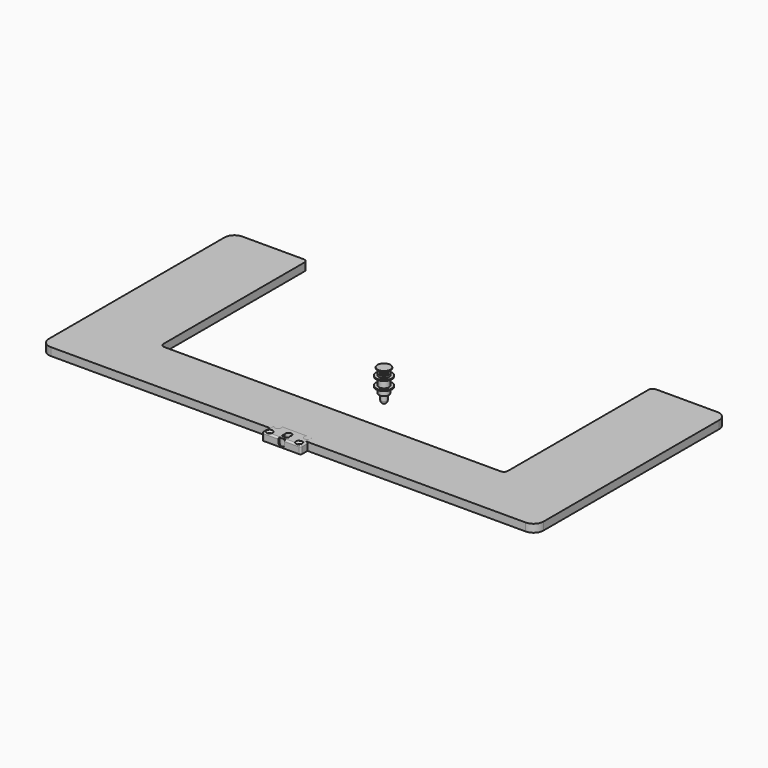
from build123d import *

# Parameters (mm, degrees)
F0_R           = 8.0391
F1_DEPTH       = 12.7
F2_W           = 62.0164461434
F2_H           = 28.0967354774
F2_R           = 4.8895
F3_DEPTH       = 12.7
F7_R           = 2.54
F9_D           = 4.7498
F9_CSINK_D     = 10.16
F9_CSINK_ANGLE = 82
F10_W          = 4.7498
F10_H          = 1.6002


with BuildPart() as f1:
    # F0 (on Top) → F1 (new body)
    with BuildSketch(Plane.XY):
        with BuildLine():
            ThreePointArc((-396.8930379433, -176.0628120543), (-392.25524501, -187.3556160105), (-381.0191923747, -192.1292588187))
            Line((-381.0191923747, -192.1292588187), (-29.9185505861, -192.1292588187))
            ThreePointArc((-29.9185505861, -192.1292588187), (-28.4575333665, -192.2996205863), (-27.0749103125, -192.801564745))
            Line((-27.0749103125, -192.801564745), (-5.7064793941, -203.503819913))
            ThreePointArc((-5.7064793941, -203.503819913), (-0.0095961873, -204.8507020685), (5.6872870194, -203.503819913))
            Line((5.6872870194, -203.503819913), (27.0557179378, -192.801564745))
            ThreePointArc((27.0557179378, -192.801564745), (28.4383409918, -192.2996205863), (29.8993582114, -192.1292588187))
            Line((29.8993582114, -192.1292588187), (381, -192.1292588187))
            ThreePointArc((381, -192.1292588187), (392.2253201513, -187.4795789701), (396.875, -176.2542588187))
            Line((396.875, -176.2542588187), (396.875, 176.1707411813))
            ThreePointArc((396.875, 176.1707411813), (392.2253201513, 187.3960613326), (381, 192.0457411813))
            Line((381, 192.0457411813), (282.575, 192.0457411813))
            ThreePointArc((282.575, 192.0457411813), (278.0848719395, 190.1858692418), (276.225, 185.6957411813))
            Line((276.225, 185.6957411813), (276.225, -96.8792588187))
            ThreePointArc((276.225, -96.8792588187), (274.3651280605, -101.3693868793), (269.875, -103.2292588187))
            Line((269.875, -103.2292588187), (-269.8930379433, -103.2292588187))
            ThreePointArc((-269.8930379433, -103.2292588187), (-274.3831660038, -101.3693868793), (-276.2430379433, -96.8792588187))
            Line((-276.2430379433, -96.8792588187), (-276.2430379433, 185.6957411813))
            ThreePointArc((-276.2430379433, 185.6957411813), (-278.1029098828, 190.1858692418), (-282.5930379433, 192.0457411813))
            Line((-282.5930379433, 192.0457411813), (-381.0180379433, 192.0457411813))
            ThreePointArc((-381.0180379433, 192.0457411813), (-392.2433580946, 187.3960613326), (-396.8930379433, 176.1707411813))
            Line((-396.8930379433, 176.1707411813), (-396.8930379433, -176.0628120543))
        make_face()
        with Locations((-0.0095961873, -192.1292588187)):
            Circle(F0_R, mode=Mode.SUBTRACT)
    extrude(amount=F1_DEPTH)


with BuildPart() as f3:
    # F2 (on Top) → F3 (new body)
    with BuildSketch(Plane.XY):
        with Locations((0, -191.5318369865)):
            Rectangle(F2_W, F2_H)
        with Locations((0, -191.5318369865)):
            Circle(F2_R, mode=Mode.SUBTRACT)
    extrude(amount=F3_DEPTH)

    # F6: sweep along a path in F4
    with BuildLine(Plane.YZ) as f6_path:
        Line((-205.5802047253, 2.0510469544), (-192.8892766759, 12.7))
    # F5 (on face) → F6 (sweep, cut)
    with BuildSketch(Plane.XZ.offset(205.5802047253)):
        with BuildLine():
            Line((-4.7625, 12.7), (-4.7625, 5.3647807799))
            ThreePointArc((-4.7625, 5.3647807799), (0, 0.6022807799), (4.7625, 5.3647807799))
            Line((4.7625, 5.3647807799), (4.7625, 12.7))
            Line((4.7625, 12.7), (-4.7625, 12.7))
        make_face()
    sweep(path=f6_path.line, mode=Mode.SUBTRACT)

    # F7
    f7_edges = [f3.edges().sort_by_distance(p)[0] for p in [
        (-31.008223, -191.531837, 12.7),
        (-17.885362, -205.580205, 12.7),
        (17.885362, -205.580205, 12.7),
        (31.008223, -191.531837, 12.7),
        (0, -177.483469, 12.7),
        (31.008223, -205.580205, 6.35),
        (31.008223, -177.483469, 6.35),
        (-31.008223, -205.580205, 6.35),
        (-31.008223, -177.483469, 6.35),
    ]]
    fillet(f7_edges, radius=F7_R)

    # F9 (through all)
    with Locations(Plane.XY.offset(12.7)):
        with Locations((-23.5967673361, -183.2025200129), (23.5967673361, -183.2025200129), (23.5967673361, -199.8611539602), (-23.5967673361, -199.8611539602)):
            CounterSinkHole(F9_D / 2, F9_CSINK_D / 2, counter_sink_angle=F9_CSINK_ANGLE)


with BuildPart() as f11:
    # F10 (on Front) → F11 (revolve)
    with BuildSketch(Plane.XZ):
        with BuildLine():
            ThreePointArc((0, -21.0152691894), (3.3675960454, -19.6203652348), (4.7625, -16.2527691894))
            Line((4.7625, -16.2527691894), (4.7625, -6.796184157))
            Line((4.7625, -6.796184157), (7.9375, -6.796184157))
            Line((7.9375, -6.796184157), (7.9375, 2.7130942824))
            Line((7.9375, 2.7130942824), (7.9375, 4.3132942824))
            Line((7.9375, 4.3132942824), (7.9375, 17.0132942824))
            Line((7.9375, 17.0132942824), (7.9375, 18.6134942824))
            Line((7.9375, 18.6134942824), (7.9375, 21.7884942824))
            Line((7.9375, 21.7884942824), (5.08, 21.7884942824))
            Line((5.08, 21.7884942824), (5.08, 23.7518632694))
            Line((5.08, 23.7518632694), (10.414, 28.596999448))
            Line((10.414, 28.596999448), (10.414, 30.1022308106))
            Line((10.414, 30.1022308106), (0, 30.1022308106))
            Line((0, 30.1022308106), (0, -21.0152691894))
        make_face()
    revolve(axis=Axis((0, 0, 4.5434808106), (0, 0, -1)))


with BuildPart() as f12:
    # F10 (on Front) → F12 (revolve)
    with BuildSketch(Plane.XZ):
        with Locations((10.3124, 17.8133942824)):
            Rectangle(F10_W, F10_H)
    revolve(axis=Axis((0, 0, 4.5434808106), (0, 0, -1)))


with BuildPart() as f12b:
    # F10 (on Front) → F12, piece 2 (revolve)
    with BuildSketch(Plane.XZ):
        with Locations((10.3124, 3.5131942824)):
            Rectangle(F10_W, F10_H)
    revolve(axis=Axis((0, 0, 4.5434808106), (0, 0, -1)))


solid = Compound([f1.part, f3.part, f11.part, f12.part, f12b.part])
